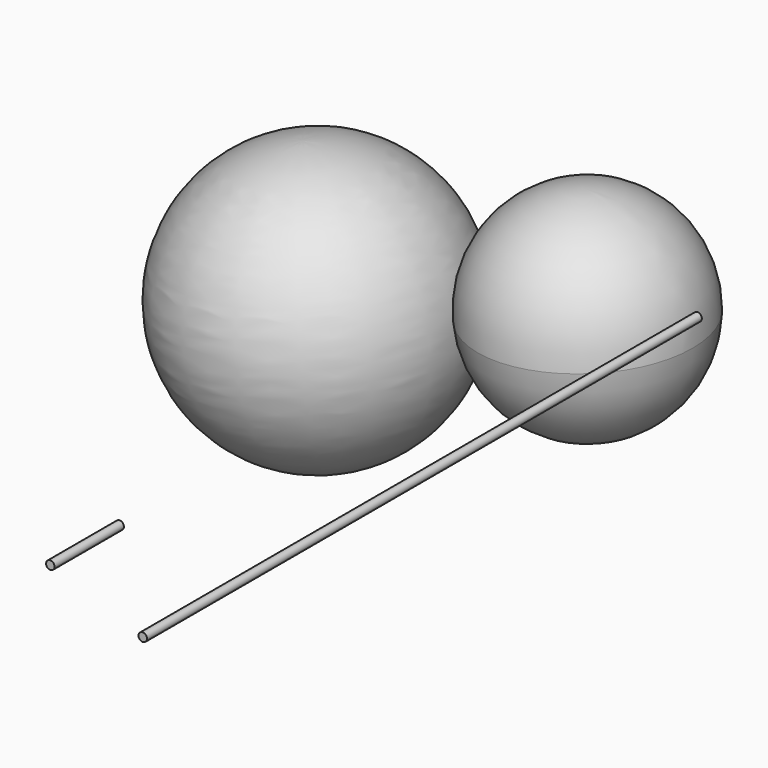
from build123d import *

# Parameters (mm, degrees)
F0_R     = 1.2446
F1_DEPTH = 203.2
F2_R     = 1.2446
F3_DEPTH = 25.4


# Not quite as in the source:
# - ends of sketch curves that miss each other by under 0.0002 mm in the source are joined


with BuildPart() as f1:
    # F0 (on Front) → F1 (new body)
    with BuildSketch(Plane.XZ):
        with Locations((-63.608661294, 25.8142799139)):
            Circle(F0_R)
    extrude(amount=F1_DEPTH)


with BuildPart() as f3:
    # F2 (on Front) → F3 (new body)
    with BuildSketch(Plane.XZ):
        with Locations((-232.9263091087, -82.9491764307)):
            Circle(F2_R)
    extrude(amount=F3_DEPTH)


with BuildPart() as f5:
    # F4 (on Front) → F5 (revolve)
    with BuildSketch(Plane.XZ):
        with BuildLine():
            Line((-179.499891461, 33.5575204974), (-170.3391089722, -45.9159741756))
            ThreePointArc((-170.3391089722, -45.9159741756), (-135.0787717268, -1.5868498537), (-179.499891461, 33.5575204974))
        make_face()
    revolve(axis=Axis((-174.9195002166, 0, -6.1792268391), (0.1145101721, 0, -0.9934220757)))


with BuildPart() as f7:
    # F6 (on Front) → F7 (revolve)
    with BuildSketch(Plane.XZ):
        with BuildLine():
            ThreePointArc((-94.4321810691, -13.5593670534), (-73.5838772535, -4.021516738), (-65.0676894112, 17.2645562973))
            ThreePointArc((-65.0676894112, 17.2645562973), (-74.6418070132, 39.6085590924), (-97.4235790279, 48.0884796481))
            Line((-97.4235790279, 48.0884796481), (-94.4321810691, -13.5593670534))
        make_face()
    revolve(axis=Axis((-95.9278800485, 0, 17.2645562973), (0.0484669391, 0, -0.9988247873)))


solid = Compound([f1.part, f3.part, f5.part, f7.part])
